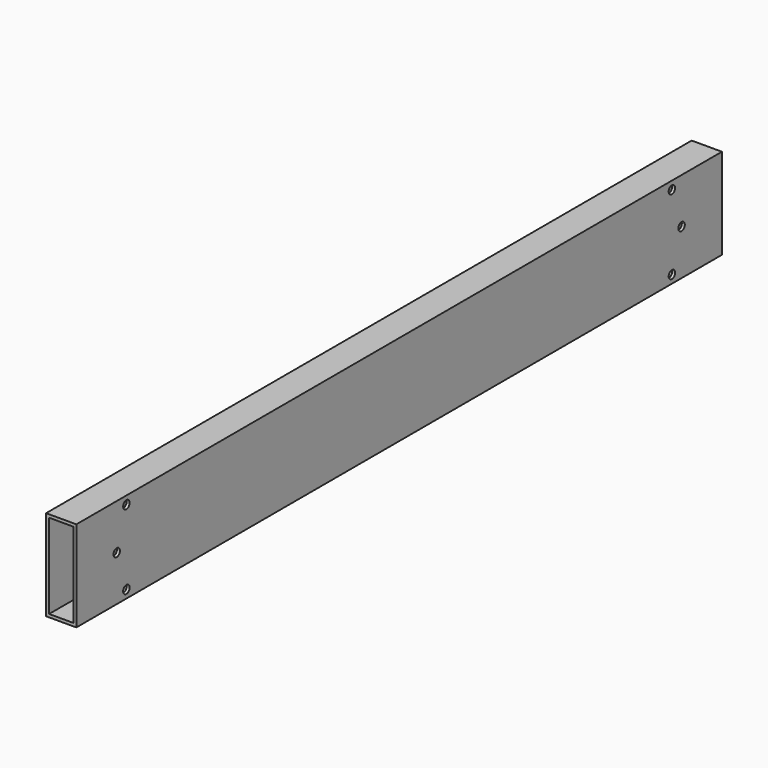
from build123d import *

# Parameters (mm, degrees)
F0_W     = 30
F0_H     = 90
F1_DEPTH = 400
F2_T     = -3
F3_R     = 4
F4_DEPTH = 30.001


# Not quite as in the source:
# - a pattern or mirror of a feature is missing from the dataset's text; its kind, count and spacing are read off the source's solid


with BuildPart() as f1:
    # F0 (on Front) → F1 (new body, symmetric)
    with BuildSketch(Plane.XZ):
        Rectangle(F0_W, F0_H)
    extrude(amount=F1_DEPTH, both=True)

    # F2
    f2_openings = [f1.faces().sort_by_distance(p)[0] for p in [
        (0, -400, 0),
        (0, 400, 0),
    ]]
    offset(amount=F2_T, openings=f2_openings)

    # F3 (on face) → F4 (cut, through all)
    with BuildSketch(Plane.YZ.offset(15)):
        with Locations((338, 37)):
            Circle(F3_R)
        with Locations((350, 0)):
            Circle(F3_R)
        with Locations((338, -37)):
            Circle(F3_R)
    f4 = extrude(amount=-F4_DEPTH, mode=Mode.SUBTRACT)

    # F4_copies: F4 across plane
    add(f4.mirror(Plane(origin=(0, 0, 0), x_dir=(0, 0, -1), z_dir=(0, -1, 0))), mode=Mode.SUBTRACT)


solid = f1.part
